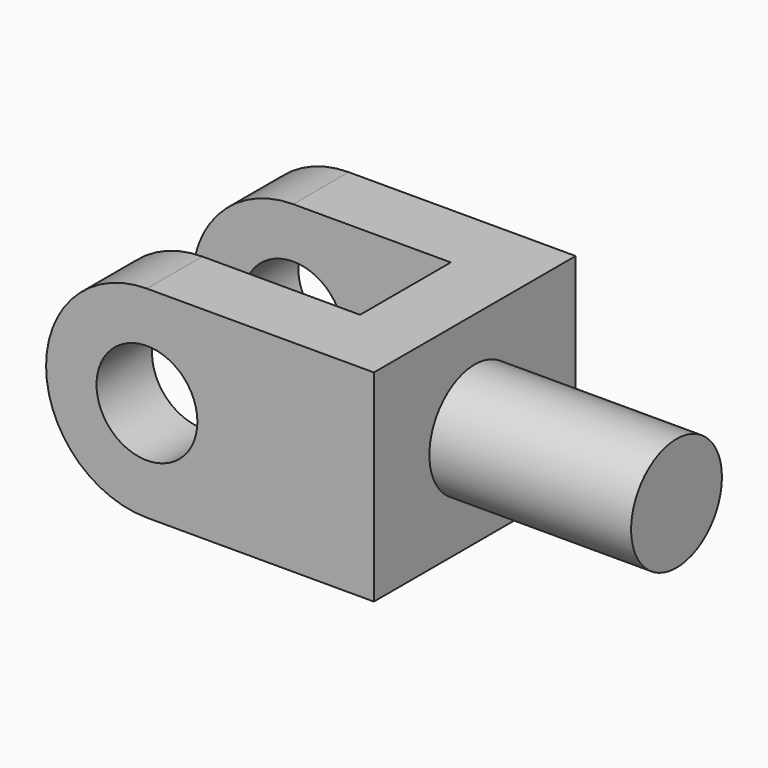
from build123d import *

# Parameters (mm, degrees)
F1_DEPTH = 812.8
F2_R     = 203.2
F3_DEPTH = 1016
F4_R     = 228.6
F5_DEPTH = 812.8
F6_R     = 406.39999
F7_R     = 406.39999


# Not quite as in the source:
# - a fillet or chamfer is up to 0.001 mm smaller than in the source, because OpenCascade refuses the exact size


with BuildPart() as f1:
    # F0 (on Top) → F1 (new body)
    with BuildSketch(Plane.XY):
        Polygon((419.8623751171, -132.2829696707), (419.8623751171, 324.9170303293), (419.8623751171, 604.3170303293), (-900.9376248829, 604.3170303293), (-900.9376248829, 324.9170303293), (140.4623751171, 324.9170303293), (140.4623751171, -132.2829696707), (-900.9376248829, -132.2829696707), (-900.9376248829, -411.6829696707), (419.8623751171, -411.6829696707), align=None)
    extrude(amount=F1_DEPTH)

    # F2 (on face) → F3 (cut)
    with BuildSketch(Plane.XZ.offset(411.6829696707)):
        with Locations((-494.5376248829, 406.4)):
            Circle(F2_R)
    extrude(amount=-F3_DEPTH, mode=Mode.SUBTRACT)

    # F4 (on face) → F5 (join)
    with BuildSketch(Plane.YZ.offset(419.8623751171)):
        with Locations((96.3170303293, 406.4)):
            Circle(F4_R)
    extrude(amount=F5_DEPTH)

    # F6 (radius 406.4 in the source; OpenCascade refuses exactly that, so slightly less here)
    f6_edges = [f1.edges().sort_by_distance(p)[0] for p in [
        (-900.937625, 464.61703, 812.8),
        (-900.937625, 464.61703, 0),
    ]]
    fillet(f6_edges, radius=F6_R)

    # F7 (radius 406.4 in the source; OpenCascade refuses exactly that, so slightly less here)
    f7_edges = [f1.edges().sort_by_distance(p)[0] for p in [
        (-900.937625, -271.98297, 812.8),
        (-900.937625, -271.98297, 0),
    ]]
    fillet(f7_edges, radius=F7_R)


solid = f1.part
